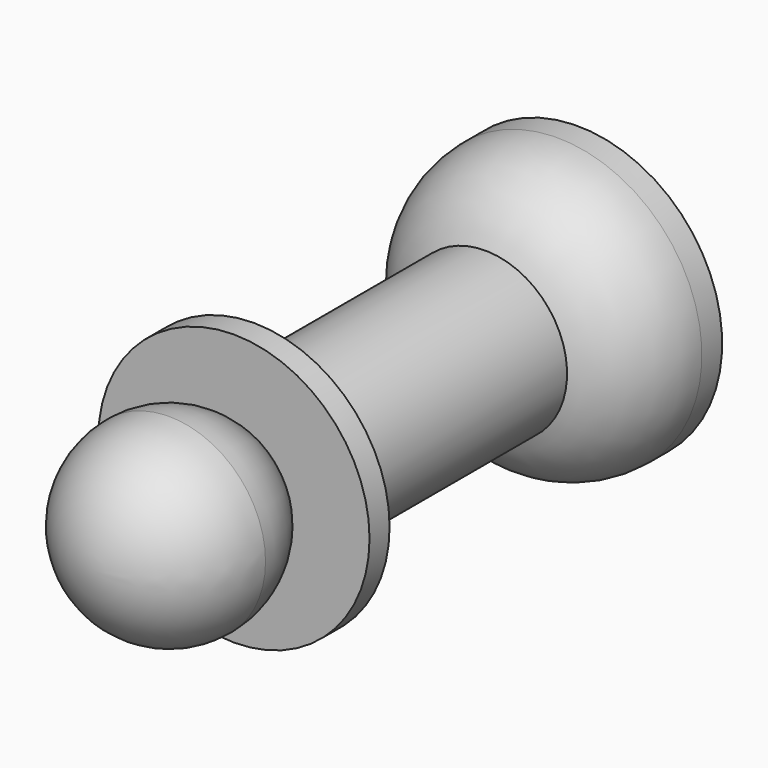
from build123d import *

# Parameters (mm, degrees)
F0_R          = 12.7
F1_DEPTH      = 25.4
F2_R          = 12.7
F3_R          = 12.69999
F4_R          = 17.8783824342
F5_DEPTH      = 1.27
F5_DEPTH_BACK = 2.032
F6_R          = 10.795
F7_DEPTH      = 38.1
F8_R          = 19.05
F9_DEPTH      = 15.24


# Not quite as in the source:
# - a fillet or chamfer that OpenCascade refuses, or shapes differently, is made with other operations: its cross-section is extruded or revolved along the edge and cut away or added
# - a fillet or chamfer is up to 0.001 mm smaller than in the source, because OpenCascade refuses the exact size


with BuildPart() as f1:
    # F0 (on Front) → F1 (new body)
    with BuildSketch(Plane.XZ):
        Circle(F0_R)
    extrude(amount=F1_DEPTH)

    # F2
    f2_edges = [f1.edges().sort_by_distance(p)[0] for p in [
        (-12.7, -25.4, 0),
    ]]
    fillet(f2_edges, radius=F2_R)

    # F3 (radius 12.7 in the source; OpenCascade refuses exactly that, so slightly less here)
    f3_edges = [f1.edges().sort_by_distance(p)[0] for p in [
        (-12.7, 0, 0),
    ]]
    fillet(f3_edges, radius=F3_R)

    # F4 (on Front) → F5 (join, two sides)
    with BuildSketch(Plane.XZ) as f5_sk:
        Circle(F4_R)
    extrude(amount=-F5_DEPTH)
    extrude(f5_sk.sketch, amount=F5_DEPTH_BACK)

    # F6 (on face) → F7 (join)
    with BuildSketch(Plane(origin=(0, 1.27, 0), x_dir=(-1, 0, 0), z_dir=(0, 1, 0))):
        Circle(F6_R)
    extrude(amount=F7_DEPTH)

    # F8 (on face) → F9 (join)
    with BuildSketch(Plane(origin=(0, 39.37, 0), x_dir=(-1, 0, 0), z_dir=(0, 1, 0))):
        Circle(F8_R)
    extrude(amount=F9_DEPTH)

    # F10: fillet of radius 12.7 on 1 edges, made by hand

    # F10_s1 → F10_t2 (revolve, cut)
    with BuildSketch(Plane.XY):
        with BuildLine():
            ThreePointArc((-19.05, 51.2667211869), (-16.7841147205, 44.0266072376), (-10.795, 39.37))
            Line((-10.795, 39.37), (-19.05, 39.37))
            Line((-19.05, 39.37), (-19.05, 51.2667211869))
        make_face()
    revolve(axis=Axis((0, 39.37, 0), (0, 1, 0)), mode=Mode.SUBTRACT)


solid = f1.part
